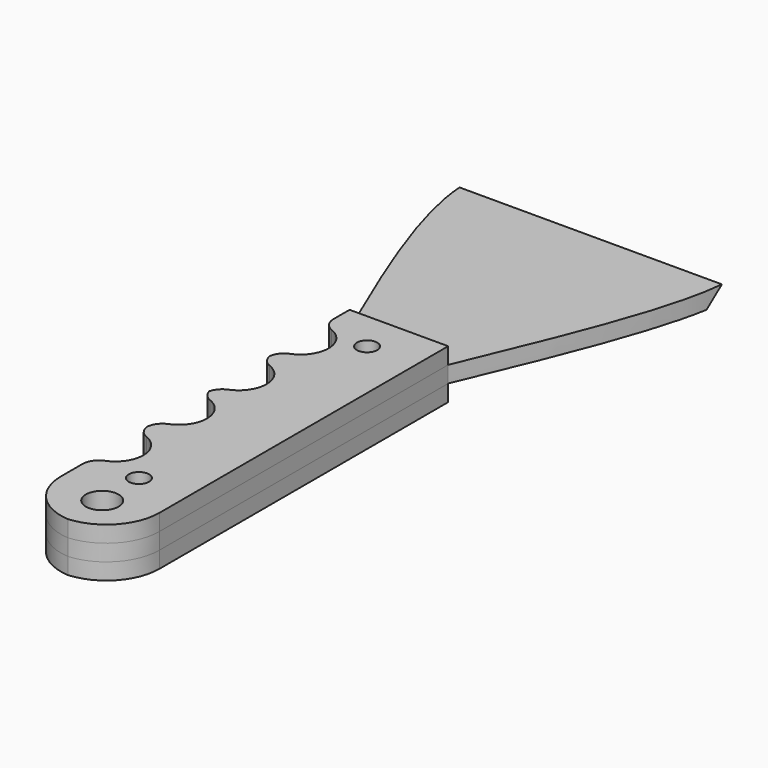
from build123d import *

# Parameters (mm, degrees)
F0_W         = 30
F0_H         = 126
F1_DEPTH     = 5
F2_T1_DEPTH  = 85.8761543395
F4_DEPTH     = 25
F5_T1_DEPTH  = 25.1996810199
F7_DEPTH     = 5
F9_DEPTH     = 5
F10_T1_DEPTH = 110.8601958556
F11_R        = 3.1
F11_R_2      = 5
F12_DEPTH    = 83.8


# Not quite as in the source:
# - a fillet or chamfer that OpenCascade refuses, or shapes differently, is made with other operations: its cross-section is extruded or revolved along the edge and cut away or added


with BuildPart() as f1:
    # F0 (on Top) → F1 (new body)
    with BuildSketch(Plane.XY):
        with BuildLine():
            add(Edge.make_bspline(
                [(1.999508217, 81.9356532991), (-10.1294136818, 110.3160546729), (-22.2583355805, 138.6964560467), (-23.000491783, 155.9356532991)],
                knots=[0, 0, 0, 0, 0.6549279326, 0.6549279326, 0.6549279326, 0.6549279326], degree=3))
            Line((1.999508217, 81.9356532991), (31.999508217, 81.9356532991))
            add(Edge.make_bspline(
                [(31.999508217, 81.9356532991), (43.8717951109, 110.1652859419), (55.7440820049, 138.3949185848), (56.999508217, 155.9356532991)],
                knots=[0, 0, 0, 0, 0.6510604818, 0.6510604818, 0.6510604818, 0.6510604818], degree=3))
            Line((56.999508217, 155.9356532991), (-23.000491783, 155.9356532991))
        make_face()
        with Locations((16.999508217, 18.9356532991)):
            Rectangle(F0_W, F0_H)
    extrude(amount=F1_DEPTH)

    # F2: fillet of radius 16.1752308679 on 2 edges, made by hand

    # F2_s2 → F2_t1 (cut)
    with BuildSketch(Plane.XY.offset(-40.4380771697)):
        with BuildLine():
            ThreePointArc((18.1747390849, -44.0643467009), (6.7371236509, -39.326731267), (1.999508217, -27.889115833))
            Line((1.999508217, -27.889115833), (1.999508217, -44.0643467009))
            Line((1.999508217, -44.0643467009), (18.1747390849, -44.0643467009))
        make_face()
        with BuildLine():
            ThreePointArc((31.999508217, -27.889115833), (27.261892783, -39.326731267), (15.8242773491, -44.0643467009))
            Line((15.8242773491, -44.0643467009), (31.999508217, -44.0643467009))
            Line((31.999508217, -44.0643467009), (31.999508217, -27.889115833))
        make_face()
    extrude(amount=F2_T1_DEPTH, mode=Mode.SUBTRACT)

    # F3 (on face) → F4 (cut)
    with BuildSketch(Plane.XY.offset(5)):
        with BuildLine():
            ThreePointArc((10.499508217, -7.1626533754), (8.0099158571, -1.1522457353), (1.999508217, 1.3373466246))
            Line((1.999508217, 1.3373466246), (1.999508217, -15.6626533754))
            ThreePointArc((1.999508217, -15.6626533754), (8.0099158571, -13.1730610155), (10.499508217, -7.1626533754))
        make_face()
        with BuildLine():
            ThreePointArc((10.499508217, 17.0258656144), (8.0099158571, 23.0362732545), (1.999508217, 25.5258656144))
            Line((1.999508217, 25.5258656144), (1.999508217, 8.5258656144))
            ThreePointArc((1.999508217, 8.5258656144), (8.0099158571, 11.0154579743), (10.499508217, 17.0258656144))
        make_face()
        with BuildLine():
            ThreePointArc((10.499508217, 39.7212654352), (8.0099158571, 45.7316730753), (1.999508217, 48.2212654352))
            Line((1.999508217, 48.2212654352), (1.999508217, 31.2212654352))
            ThreePointArc((1.999508217, 31.2212654352), (8.0099158571, 33.7108577951), (10.499508217, 39.7212654352))
        make_face()
        with BuildLine():
            ThreePointArc((1.999508217, 54.8125379682), (8.0099158571, 57.3021303281), (10.499508217, 63.3125379682))
            ThreePointArc((10.499508217, 63.3125379682), (8.0099158571, 69.3229456082), (1.999508217, 71.8125379682))
            Line((1.999508217, 71.8125379682), (1.999508217, 54.8125379682))
        make_face()
    extrude(amount=-F4_DEPTH, mode=Mode.SUBTRACT)

    # F5: fillet of radius 5 on 8 edges, made by hand

    # F5_s2 → F5_t1 (cut)
    with BuildSketch(Plane.XY.offset(-10.09984051)):
        with BuildLine():
            ThreePointArc((5.1476563651, -15.0581687631), (2.8607125432, -16.897171541), (1.999508217, -19.7025895794))
            Line((1.999508217, -19.7025895794), (1.999508217, -15.6626533754))
            ThreePointArc((1.999508217, -15.6626533754), (3.6023368423, -15.5101644055), (5.1476563651, -15.0581687631))
        make_face()
        with BuildLine():
            ThreePointArc((1.999508217, 5.3772828286), (2.8607125432, 2.5718647901), (5.1476563651, 0.7328620123))
            ThreePointArc((5.1476563651, 0.7328620123), (3.6023368423, 1.1848576547), (1.999508217, 1.3373466246))
            Line((1.999508217, 1.3373466246), (1.999508217, 5.3772828286))
        make_face()
        with BuildLine():
            ThreePointArc((5.1476563651, 9.1303502267), (2.8607125432, 7.2913474489), (1.999508217, 4.4859294104))
            Line((1.999508217, 4.4859294104), (1.999508217, 8.5258656144))
            ThreePointArc((1.999508217, 8.5258656144), (3.6023368423, 8.6783545843), (5.1476563651, 9.1303502267))
        make_face()
        with BuildLine():
            ThreePointArc((1.999508217, 29.5658018184), (2.8607125432, 26.76038378), (5.1476563651, 24.9213810021))
            ThreePointArc((5.1476563651, 24.9213810021), (3.6023368423, 25.3733766445), (1.999508217, 25.5258656144))
            Line((1.999508217, 25.5258656144), (1.999508217, 29.5658018184))
        make_face()
        with BuildLine():
            ThreePointArc((5.1476563651, 31.8257500475), (2.8607125432, 29.9867472697), (1.999508217, 27.1813292312))
            Line((1.999508217, 27.1813292312), (1.999508217, 31.2212654352))
            ThreePointArc((1.999508217, 31.2212654352), (3.6023368423, 31.3737544051), (5.1476563651, 31.8257500475))
        make_face()
        with BuildLine():
            ThreePointArc((1.999508217, 52.2612016392), (2.8607125432, 49.4557836008), (5.1476563651, 47.6167808229))
            ThreePointArc((5.1476563651, 47.6167808229), (3.6023368423, 48.0687764653), (1.999508217, 48.2212654352))
            Line((1.999508217, 48.2212654352), (1.999508217, 52.2612016392))
        make_face()
        with BuildLine():
            ThreePointArc((5.1476563651, 55.4170225805), (2.8607125432, 53.5780198026), (1.999508217, 50.7726017642))
            Line((1.999508217, 50.7726017642), (1.999508217, 54.8125379682))
            ThreePointArc((1.999508217, 54.8125379682), (3.6023368423, 54.9650269381), (5.1476563651, 55.4170225805))
        make_face()
        with BuildLine():
            ThreePointArc((1.999508217, 75.8524741721), (2.8607125432, 73.0470561337), (5.1476563651, 71.2080533559))
            ThreePointArc((5.1476563651, 71.2080533559), (3.6023368423, 71.6600489983), (1.999508217, 71.8125379682))
            Line((1.999508217, 71.8125379682), (1.999508217, 75.8524741721))
        make_face()
    extrude(amount=F5_T1_DEPTH, mode=Mode.SUBTRACT)

    # F10: chamfer of 6 on 1 edges, made by hand

    # F10_s2 → F10_t1 (cut)
    with BuildSketch(Plane.YZ.offset(-38.4305897108)):
        Polygon((155.9356532991, 6), (149.9356532991, 0), (155.9356532991, 0), align=None)
    extrude(amount=F10_T1_DEPTH, mode=Mode.SUBTRACT)


with BuildPart() as f7:
    # F6 (on face) → F7 (new body)
    with BuildSketch(Plane.XY.offset(5)):
        with BuildLine():
            Line((31.999508217, 81.9356532991), (1.999508217, 81.9356532991))
            Line((1.999508217, 81.9356532991), (1.999508217, 75.8524741721))
            ThreePointArc((1.999508217, 75.8524741721), (2.8607125432, 73.0470561337), (5.1476563651, 71.2080533559))
            ThreePointArc((5.1476563651, 71.2080533559), (10.499508217, 63.3125379682), (5.1476563651, 55.4170225805))
            ThreePointArc((5.1476563651, 55.4170225805), (3.0816482724, 53.8791067866), (2.0552168014, 51.5169017017))
            ThreePointArc((2.0552168014, 51.5169017017), (3.0816482724, 49.1546966168), (5.1476563651, 47.6167808229))
            ThreePointArc((5.1476563651, 47.6167808229), (10.499508217, 39.7212654352), (5.1476563651, 31.8257500475))
            ThreePointArc((5.1476563651, 31.8257500475), (3.227576814, 30.4634830197), (2.1437309754, 28.3735655249))
            ThreePointArc((2.1437309754, 28.3735655249), (3.227576814, 26.2836480299), (5.1476563651, 24.9213810021))
            ThreePointArc((5.1476563651, 24.9213810021), (10.499508217, 17.0258656144), (5.1476563651, 9.1303502267))
            ThreePointArc((5.1476563651, 9.1303502267), (2.989988744, 7.4731946473), (2.0194106004, 4.9316061195))
            ThreePointArc((2.0194106004, 4.9316061195), (2.989988744, 2.3900175917), (5.1476563651, 0.7328620123))
            ThreePointArc((5.1476563651, 0.7328620123), (10.499508217, -7.1626533754), (5.1476563651, -15.0581687631))
            ThreePointArc((5.1476563651, -15.0581687631), (2.8607125432, -16.897171541), (1.999508217, -19.7025895794))
            Line((1.999508217, -19.7025895794), (1.999508217, -27.889115833))
            ThreePointArc((1.999508217, -27.889115833), (6.3289017518, -38.9033898222), (16.9995082169, -44.0215963006))
            ThreePointArc((16.9995082169, -44.0215963006), (27.6701146821, -38.9033898222), (31.999508217, -27.889115833))
            Line((31.999508217, -27.889115833), (31.999508217, 81.9356532991))
        make_face()
    extrude(amount=F7_DEPTH)


with BuildPart() as f9:
    # F8 (on face) → F9 (new body)
    with BuildSketch(Plane(origin=(0, 0, 0), x_dir=(1, 0, 0), z_dir=(0, 0, -1))):
        with BuildLine():
            Line((1.999508217, -75.8524741721), (1.999508217, -81.9356532991))
            Line((1.999508217, -81.9356532991), (31.999508217, -81.9356532991))
            Line((31.999508217, -81.9356532991), (31.999508217, 27.889115833))
            ThreePointArc((31.999508217, 27.889115833), (27.6701146821, 38.9033898222), (16.9995082169, 44.0215963006))
            ThreePointArc((16.9995082169, 44.0215963006), (6.3289017518, 38.9033898222), (1.999508217, 27.889115833))
            Line((1.999508217, 27.889115833), (1.999508217, 19.7025895794))
            ThreePointArc((1.999508217, 19.7025895794), (2.8607125432, 16.897171541), (5.1476563651, 15.0581687631))
            ThreePointArc((5.1476563651, 15.0581687631), (10.499508217, 7.1626533754), (5.1476563651, -0.7328620123))
            ThreePointArc((5.1476563651, -0.7328620123), (2.989988744, -2.3900175917), (2.0194106004, -4.9316061195))
            ThreePointArc((2.0194106004, -4.9316061195), (2.989988744, -7.4731946473), (5.1476563651, -9.1303502267))
            ThreePointArc((5.1476563651, -9.1303502267), (10.499508217, -17.0258656144), (5.1476563651, -24.9213810021))
            ThreePointArc((5.1476563651, -24.9213810021), (3.227576814, -26.2836480299), (2.1437309754, -28.3735655249))
            ThreePointArc((2.1437309754, -28.3735655249), (3.227576814, -30.4634830197), (5.1476563651, -31.8257500475))
            ThreePointArc((5.1476563651, -31.8257500475), (10.499508217, -39.7212654352), (5.1476563651, -47.6167808229))
            ThreePointArc((5.1476563651, -47.6167808229), (3.0816482724, -49.1546966168), (2.0552168014, -51.5169017017))
            ThreePointArc((2.0552168014, -51.5169017017), (3.0816482724, -53.8791067866), (5.1476563651, -55.4170225805))
            ThreePointArc((5.1476563651, -55.4170225805), (10.499508217, -63.3125379682), (5.1476563651, -71.2080533559))
            ThreePointArc((5.1476563651, -71.2080533559), (2.8607125432, -73.0470561337), (1.999508217, -75.8524741721))
        make_face()
    extrude(amount=F9_DEPTH)


with BuildPart() as f12_tool:
    # F11 (on face) → F12 (new body)
    with BuildSketch(Plane(origin=(0, 0, -5), x_dir=(1, 0, 0), z_dir=(0, 0, -1))):
        with Locations((16.999508217, -69.8356532991)):
            Circle(F11_R)
        with Locations((16.999508217, 16.9651284814)):
            Circle(F11_R)
        with Locations((17.429100106, 31.4532717611)):
            Circle(F11_R_2)
    extrude(amount=-F12_DEPTH)


with BuildPart() as f1_1:
    add(f1.part)

    # F12: cut by f12_tool
    add(f12_tool.part, mode=Mode.SUBTRACT)


with BuildPart() as f7_1:
    add(f7.part)

    # F12: cut by f12_tool
    add(f12_tool.part, mode=Mode.SUBTRACT)


with BuildPart() as f9_1:
    add(f9.part)

    # F12: cut by f12_tool
    add(f12_tool.part, mode=Mode.SUBTRACT)


solid = Compound([f1_1.part, f7_1.part, f9_1.part])
